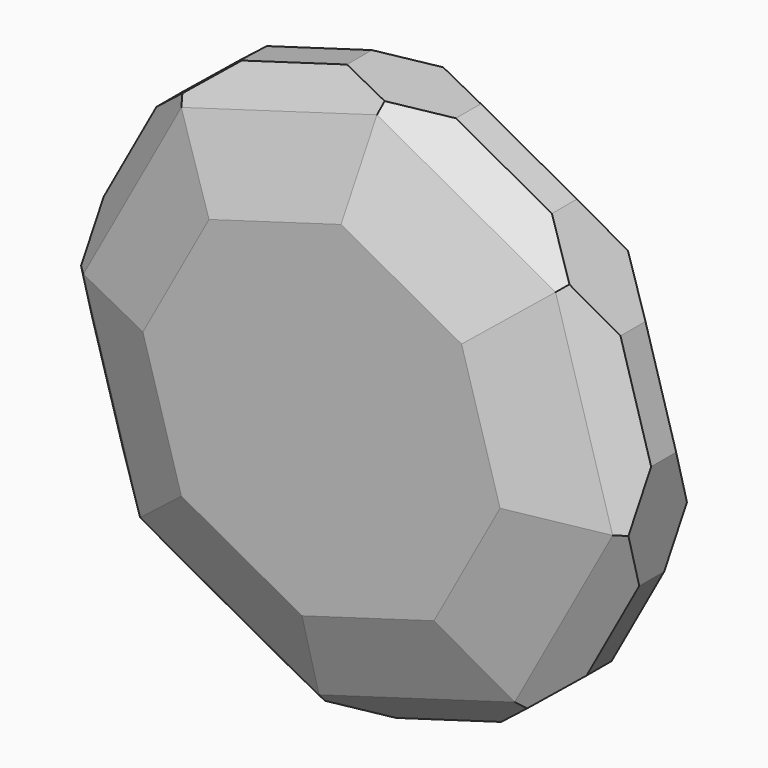
from build123d import *

# Parameters (mm, degrees)
F1_DEPTH = 25.4
F2_SIZE  = 10.16
F3_SIZE  = 7.62
F4_SIZE  = 7.62
F5_SIZE  = 10.16
F6_SIZE  = 7.62


with BuildPart() as f1:
    # F0 (on Front) → F1 (new body)
    with BuildSketch(Plane.XZ):
        Polygon((40.479728647, 21.0820164172), (29.3306543749, 34.9681649717), (13.7162538572, 43.5307273965), (-3.986321972, 45.4661311822), (-21.0820164172, 40.479728647), (-34.9681649717, 29.3306543749), (-43.5307273965, 13.7162538572), (-45.4661311822, -3.986321972), (-40.479728647, -21.0820164172), (-29.3306543749, -34.9681649717), (-13.7162538572, -43.5307273965), (3.986321972, -45.4661311822), (21.0820164172, -40.479728647), (34.9681649717, -29.3306543749), (43.5307273965, -13.7162538572), (45.4661311822, 3.986321972), align=None)
    extrude(amount=F1_DEPTH)

    # F2 (call 1 of 8: OpenCascade refuses the feature's edges together)
    f2_edges = [f1.edges().sort_by_distance(p)[0] for p in [
        (39.249446, -25.4, -21.523454),
    ]]
    chamfer(f2_edges, length=F2_SIZE)

    # F2#2 (call 2 of 8)
    f2_2_edges = [f1.edges().sort_by_distance(p)[0] for p in [
        (42.97293, -25.4, 12.534169),
    ]]
    chamfer(f2_2_edges, length=F2_SIZE)

    # F2#3 (call 3 of 8)
    f2_3_edges = [f1.edges().sort_by_distance(p)[0] for p in [
        (21.523454, -25.4, 39.249446),
    ]]
    chamfer(f2_3_edges, length=F2_SIZE)

    # F2#4 (call 4 of 8)
    f2_4_edges = [f1.edges().sort_by_distance(p)[0] for p in [
        (-12.534169, -25.4, 42.97293),
    ]]
    chamfer(f2_4_edges, length=F2_SIZE)

    # F2#5 (call 5 of 8)
    f2_5_edges = [f1.edges().sort_by_distance(p)[0] for p in [
        (-39.249446, -25.4, 21.523454),
    ]]
    chamfer(f2_5_edges, length=F2_SIZE)

    # F2#6 (call 6 of 8)
    f2_6_edges = [f1.edges().sort_by_distance(p)[0] for p in [
        (-42.97293, -25.4, -12.534169),
    ]]
    chamfer(f2_6_edges, length=F2_SIZE)

    # F2#7 (call 7 of 8)
    f2_7_edges = [f1.edges().sort_by_distance(p)[0] for p in [
        (-21.523454, -25.4, -39.249446),
    ]]
    chamfer(f2_7_edges, length=F2_SIZE)

    # F2#8 (call 8 of 8)
    f2_8_edges = [f1.edges().sort_by_distance(p)[0] for p in [
        (12.534169, -25.4, -42.97293),
    ]]
    chamfer(f2_8_edges, length=F2_SIZE)

    # F3
    f3_edges = [f1.edges().sort_by_distance(p)[0] for p in [
        (-30.34099, -25.4, 16.638271),
        (16.638271, -25.4, 30.34099),
        (30.34099, -25.4, -16.638271),
        (-16.638271, -25.4, -30.34099),
    ]]
    chamfer(f3_edges, length=F3_SIZE)

    # F4
    f4_edges = [f1.edges().sort_by_distance(p)[0] for p in [
        (-9.689286, -25.4, 33.219354),
        (33.219354, -25.4, 9.689286),
        (9.689286, -25.4, -33.219354),
        (-33.219354, -25.4, -9.689286),
    ]]
    chamfer(f4_edges, length=F4_SIZE)

    # F5 (call 1 of 8: OpenCascade refuses the feature's edges together)
    f5_edges = [f1.edges().sort_by_distance(p)[0] for p in [
        (-21.523454, 0, -39.249446),
    ]]
    chamfer(f5_edges, length=F5_SIZE)

    # F5#2 (call 2 of 8)
    f5_2_edges = [f1.edges().sort_by_distance(p)[0] for p in [
        (12.534169, 0, -42.97293),
    ]]
    chamfer(f5_2_edges, length=F5_SIZE)

    # F5#3 (call 3 of 8)
    f5_3_edges = [f1.edges().sort_by_distance(p)[0] for p in [
        (39.249446, 0, -21.523454),
    ]]
    chamfer(f5_3_edges, length=F5_SIZE)

    # F5#4 (call 4 of 8)
    f5_4_edges = [f1.edges().sort_by_distance(p)[0] for p in [
        (42.97293, 0, 12.534169),
    ]]
    chamfer(f5_4_edges, length=F5_SIZE)

    # F5#5 (call 5 of 8)
    f5_5_edges = [f1.edges().sort_by_distance(p)[0] for p in [
        (21.523454, 0, 39.249446),
    ]]
    chamfer(f5_5_edges, length=F5_SIZE)

    # F5#6 (call 6 of 8)
    f5_6_edges = [f1.edges().sort_by_distance(p)[0] for p in [
        (-12.534169, 0, 42.97293),
    ]]
    chamfer(f5_6_edges, length=F5_SIZE)

    # F5#7 (call 7 of 8)
    f5_7_edges = [f1.edges().sort_by_distance(p)[0] for p in [
        (-39.249446, 0, 21.523454),
    ]]
    chamfer(f5_7_edges, length=F5_SIZE)

    # F5#8 (call 8 of 8)
    f5_8_edges = [f1.edges().sort_by_distance(p)[0] for p in [
        (-42.97293, 0, -12.534169),
    ]]
    chamfer(f5_8_edges, length=F5_SIZE)

    # F6
    f6_edges = [f1.edges().sort_by_distance(p)[0] for p in [
        (16.638271, 0, 30.34099),
        (-9.689286, 0, 33.219354),
        (-30.34099, 0, 16.638271),
        (-33.219354, 0, -9.689286),
        (-16.638271, 0, -30.34099),
        (9.689286, 0, -33.219354),
        (30.34099, 0, -16.638271),
        (33.219354, 0, 9.689286),
    ]]
    chamfer(f6_edges, length=F6_SIZE)


solid = f1.part
